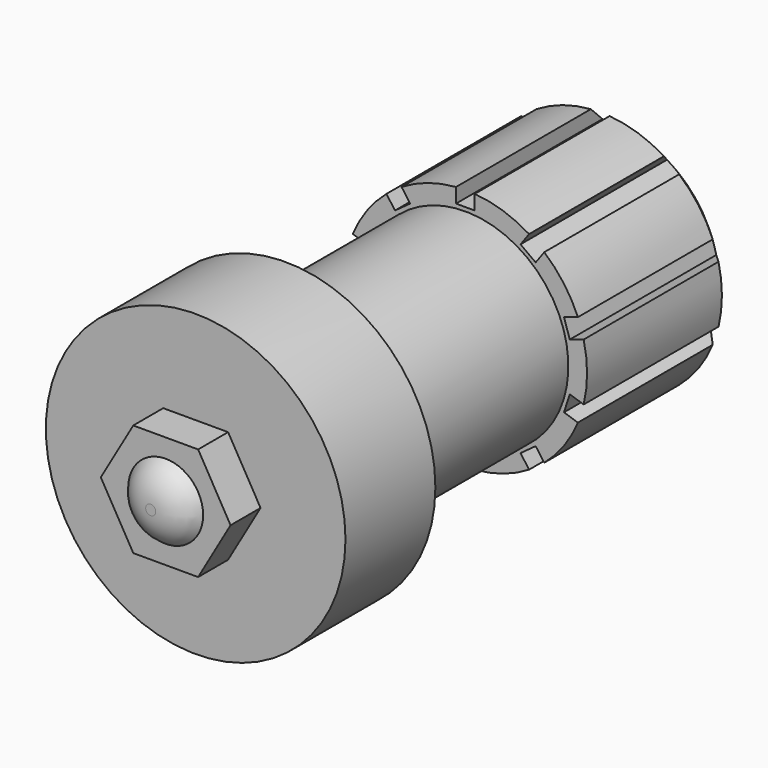
from build123d import *

# Parameters (mm, degrees)
F0_R             = 8
F1_DEPTH         = 6
F3_DEPTH         = 2
F4_R             = 2
F5_DEPTH         = 1
F7_R             = 5.5
F8_DEPTH         = 22
F9_R             = 6.5
F9_R_2           = 5.5
F10_DEPTH        = 10
F11_SIZE         = 1
F12_W            = 1
F12_H            = 2
F13_DEPTH        = 20
F13_COPIES_COUNT = 10


# Not quite as in the source:
# - a fillet or chamfer that OpenCascade refuses, or shapes differently, is made with other operations: its cross-section is extruded or revolved along the edge and cut away or added
# - a pattern or mirror of a feature is missing from the dataset's text; its kind, count and spacing are read off the source's solid


with BuildPart() as f1:
    # F0 (on Front) → F1 (new body)
    with BuildSketch(Plane.XZ):
        Circle(F0_R)
    extrude(amount=-F1_DEPTH)

    # F2 (on face) → F3 (join)
    with BuildSketch(Plane.XZ):
        Polygon((1.7320508076, 3), (-1.7320508076, 3), (-3.4641016151, 0), (-1.7320508076, -3), (1.7320508076, -3), (3.4641016151, 0), align=None)
    extrude(amount=F3_DEPTH)

    # F4 (on face) → F5 (join)
    with BuildSketch(Plane.XZ.offset(2)):
        Circle(F4_R)
    extrude(amount=F5_DEPTH)

    # F6: fillet of radius 2 on 1 edges, made by hand

    # F6_s1 → F6_t2 (revolve, cut)
    with BuildSketch(Plane.XY):
        with BuildLine():
            ThreePointArc((2, -2), (1.2679491924, -2.7320508076), (0.2679491924, -3))
            Line((0.2679491924, -3), (2, -3))
            Line((2, -3), (2, -2))
        make_face()
    revolve(axis=Axis((0, -3, 0), (0, -1, 0)), mode=Mode.SUBTRACT)

    # F7 (on face) → F8 (join)
    with BuildSketch(Plane(origin=(0, 6, 0), x_dir=(-1, 0, 0), z_dir=(0, 1, 0))):
        Circle(F7_R)
    extrude(amount=F8_DEPTH)

    # F9 (on face) → F10 (join)
    with BuildSketch(Plane(origin=(0, 28, 0), x_dir=(-1, 0, 0), z_dir=(0, 1, 0))):
        Circle(F9_R)
        Circle(F9_R_2, mode=Mode.SUBTRACT)
    extrude(amount=-F10_DEPTH)

    # F11
    f11_edges = [f1.edges().sort_by_distance(p)[0] for p in [
        (6.5, 28, 0),
    ]]
    chamfer(f11_edges, length=F11_SIZE)

    # F12 (on face) → F13 (cut)
    with BuildSketch(Plane(origin=(0, 28, 0), x_dir=(-1, 0, 0), z_dir=(0, 1, 0))):
        with Locations((0, 6.7)):
            Rectangle(F12_W, F12_H)
    f13 = extrude(amount=-F13_DEPTH, mode=Mode.SUBTRACT)

    # F13_copies: F13 ×10 about axis
    f13_copies_axis = Axis((0, 0, 0), (0, 1, 0))
    for i in range(1, F13_COPIES_COUNT):
        add(f13.rotate(f13_copies_axis, i * 360 / F13_COPIES_COUNT), mode=Mode.SUBTRACT)


solid = f1.part
